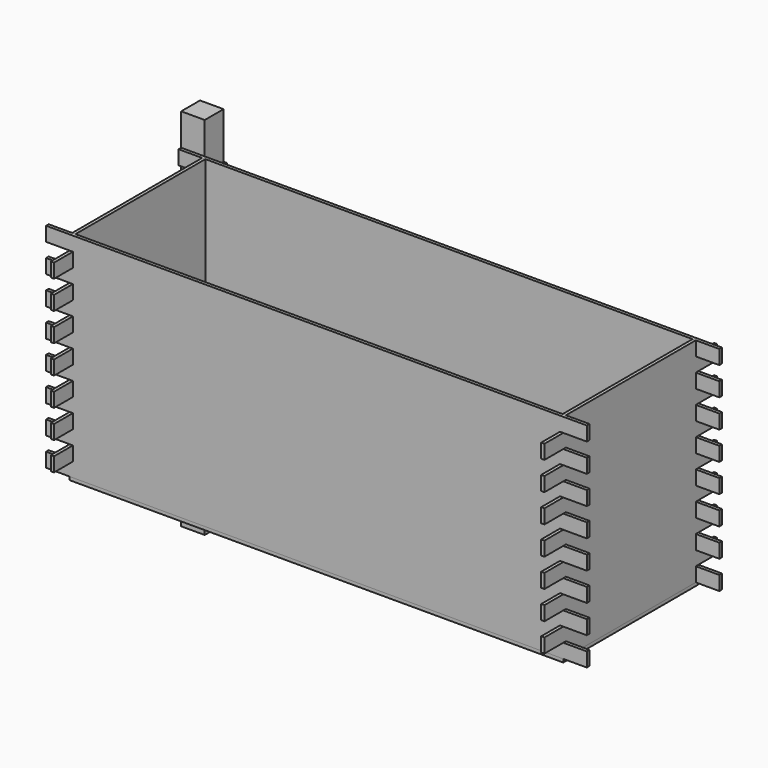
from build123d import *

# Parameters (mm, degrees)
F1_DEPTH  = 8
F3_DEPTH  = 8
F8_DEPTH  = 8
F11_DEPTH = 8
F12_W     = 1216
F12_H     = 416
F13_DEPTH = 8
F14_W     = 1200
F14_H     = 400
F15_DEPTH = 4
F17_W     = 58
F17_H     = 58
F18_DEPTH = 900


# Not quite as in the source:
# - a feature names something its author has since deleted; it is built from what else it names


with BuildPart() as f1:
    # F0 (on Front) → F1 (new body)
    with BuildSketch(Plane.XZ):
        Polygon((600, 262.5), (-600, 262.5), (-666, 262.5), (-666, 227.5), (-600, 227.5), (-600, 192.5), (-666, 192.5), (-666, 157.5), (-600, 157.5), (-600, 122.5), (-666, 122.5), (-666, 87.5), (-600, 87.5), (-600, 52.5), (-666, 52.5), (-666, 17.5), (-600, 17.5), (-600, -17.5), (-666, -17.5), (-666, -52.5), (-600, -52.5), (-600, -87.5), (-666, -87.5), (-666, -122.5), (-600, -122.5), (-600, -157.5), (-666, -157.5), (-666, -192.5), (-600, -192.5), (-600, -227.5), (-666, -227.5), (-666, -262.5), (-600, -262.5), (600, -262.5), (666, -262.5), (666, -227.5), (600, -227.5), (600, -192.5), (666, -192.5), (666, -157.5), (600, -157.5), (600, -122.5), (666, -122.5), (666, -87.5), (600, -87.5), (600, -52.5), (666, -52.5), (666, -17.5), (600, -17.5), (600, 17.5), (666, 17.5), (666, 52.5), (600, 52.5), (600, 87.5), (666, 87.5), (666, 122.5), (600, 122.5), (600, 157.5), (666, 157.5), (666, 192.5), (600, 192.5), (600, 227.5), (666, 227.5), (666, 262.5), align=None)
    extrude(amount=F1_DEPTH)


with BuildPart() as f3:
    # F2 (on face) → F3 (new body)
    with BuildSketch(Plane(origin=(-600, 0, 0), x_dir=(0, -1, 0), z_dir=(-1, 0, 0))):
        Polygon((0, 227.5), (0, 262.5), (-200, 262.5), (-400, 262.5), (-400, 227.5), (-466, 227.5), (-466, 192.5), (-400, 192.5), (-400, 157.5), (-466, 157.5), (-466, 122.5), (-400, 122.5), (-400, 87.5), (-466, 87.5), (-466, 52.5), (-400, 52.5), (-400, 17.5), (-466, 17.5), (-466, -17.5), (-400, -17.5), (-400, -52.5), (-466, -52.5), (-466, -87.5), (-400, -87.5), (-400, -122.5), (-466, -122.5), (-466, -157.5), (-400, -157.5), (-400, -192.5), (-466, -192.5), (-466, -227.5), (-400, -227.5), (-400, -262.5), (-200, -262.5), (0, -262.5), (0, -227.5), (66, -227.5), (66, -192.5), (0, -192.5), (0, -157.5), (66, -157.5), (66, -122.5), (0, -122.5), (0, -87.5), (66, -87.5), (66, -52.5), (0, -52.5), (0, -17.5), (66, -17.5), (66, 17.5), (0, 17.5), (0, 52.5), (66, 52.5), (66, 87.5), (0, 87.5), (0, 122.5), (66, 122.5), (66, 157.5), (0, 157.5), (0, 192.5), (66, 192.5), (66, 227.5), align=None)
    extrude(amount=F3_DEPTH)


with BuildPart() as f4_1:
    # F4: copy of F1
    add(f1.part.moved(Location((0, 408, 0))))


with BuildPart() as f5_1:
    # F5: copy of F3
    add(f3.part.moved(Location((1208, 0, 0))))


with BuildPart() as f8:
    # F7 (on face) → F8 (new body)
    with BuildSketch(Plane(origin=(0, 400, 0), x_dir=(-1, 0, 0), z_dir=(0, 1, 0))):
        Polygon((-666, -227.5), (-666, -262.5), (666, -262.5), (666, -227.5), (600, -227.5), (600, -192.5), (666, -192.5), (666, -157.5), (600, -157.5), (600, -122.5), (666, -122.5), (666, -87.5), (600, -87.5), (600, -52.5), (666, -52.5), (666, -17.5), (600, -17.5), (600, 17.5), (666, 17.5), (666, 52.5), (600, 52.5), (600, 87.5), (666, 87.5), (666, 122.5), (600, 122.5), (600, 157.5), (666, 157.5), (666, 192.5), (600, 192.5), (600, 227.5), (666, 227.5), (666, 262.5), (-666, 262.5), (-666, 227.5), (-600, 227.5), (-600, 192.5), (-666, 192.5), (-666, 157.5), (-600, 157.5), (-600, 122.5), (-666, 122.5), (-666, 87.5), (-600, 87.5), (-600, 52.5), (-666, 52.5), (-666, 17.5), (-600, 17.5), (-600, -17.5), (-666, -17.5), (-666, -52.5), (-600, -52.5), (-600, -87.5), (-666, -87.5), (-666, -122.5), (-600, -122.5), (-600, -157.5), (-666, -157.5), (-666, -192.5), (-600, -192.5), (-600, -227.5), align=None)
    extrude(amount=F8_DEPTH)


with BuildPart() as f11:
    # F10 (on face) → F11 (new body)
    with BuildSketch(Plane.YZ.offset(600)):
        Polygon((-66, 192.5), (0, 192.5), (0, 157.5), (-66, 157.5), (-66, 122.5), (0, 122.5), (0, 87.5), (-66, 87.5), (-66, 52.5), (0, 52.5), (0, 17.5), (-66, 17.5), (-66, -17.5), (0, -17.5), (0, -52.5), (-66, -52.5), (-66, -87.5), (0, -87.5), (0, -122.5), (-66, -122.5), (-66, -157.5), (0, -157.5), (0, -192.5), (-66, -192.5), (-66, -227.5), (0, -227.5), (0, -262.5), (400, -262.5), (400, -227.5), (466, -227.5), (466, -192.5), (400, -192.5), (400, -157.5), (466, -157.5), (466, -122.5), (400, -122.5), (400, -87.5), (466, -87.5), (466, -52.5), (400, -52.5), (400, -17.5), (466, -17.5), (466, 17.5), (400, 17.5), (400, 52.5), (466, 52.5), (466, 87.5), (400, 87.5), (400, 122.5), (466, 122.5), (466, 157.5), (400, 157.5), (400, 192.5), (466, 192.5), (466, 227.5), (400, 227.5), (400, 262.5), (0, 262.5), (0, 227.5), (-66, 227.5), align=None)
    extrude(amount=F11_DEPTH)


with BuildPart() as f13:
    # F12 (on face) → F13 (new body)
    with BuildSketch(Plane(origin=(0, 0, -262.5), x_dir=(1, 0, 0), z_dir=(0, 0, -1))):
        with Locations((0, -200)):
            Rectangle(F12_W, F12_H)
    extrude(amount=F13_DEPTH)

    # F14 (on face) → F15 (join)
    with BuildSketch(Plane.XY.offset(-262.5)):
        with Locations((0, 200)):
            Rectangle(F14_W, F14_H)
    extrude(amount=F15_DEPTH)


with BuildPart() as f18:
    # F17 (on offset) → F18 (new body)
    with BuildSketch(Plane.XY.offset(341.5)):
        with Locations((-637, 437)):
            Rectangle(F17_W, F17_H)
    extrude(amount=-F18_DEPTH)


solid = Compound([f1.part, f3.part, f8.part, f11.part, f13.part, f18.part])
